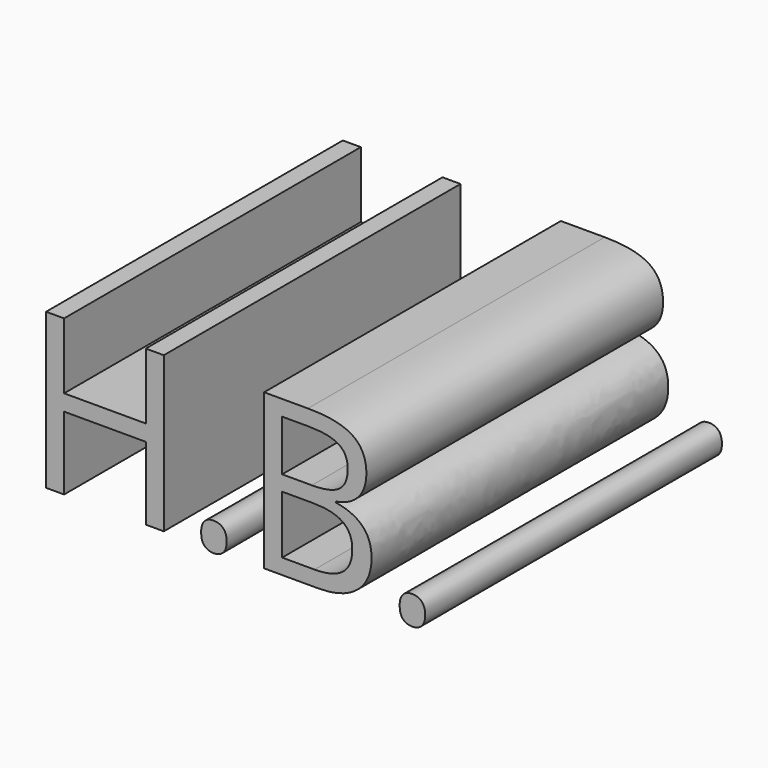
from build123d import *

# Parameters (mm, degrees)
F1_TEXT_SIZE = 3.1234511375
F2_DEPTH     = 5.334


# Not quite as in the source:
# - Text() gives the source's letters only with a copy of the font that has no kerning and outlines rounded to 1/6400 em; it was checked with that copy


with BuildPart() as f2:
    # F1 (on face) → F2 (new body)
    with BuildSketch(Plane.XZ):
        with Locations((-29.7670699656, -1.3008281821)):
            Text('H.B.', F1_TEXT_SIZE, font='Open Sans', text_align=(TextAlign.LEFT, TextAlign.BOTTOM))
    extrude(amount=F2_DEPTH)


solid = f2.part
